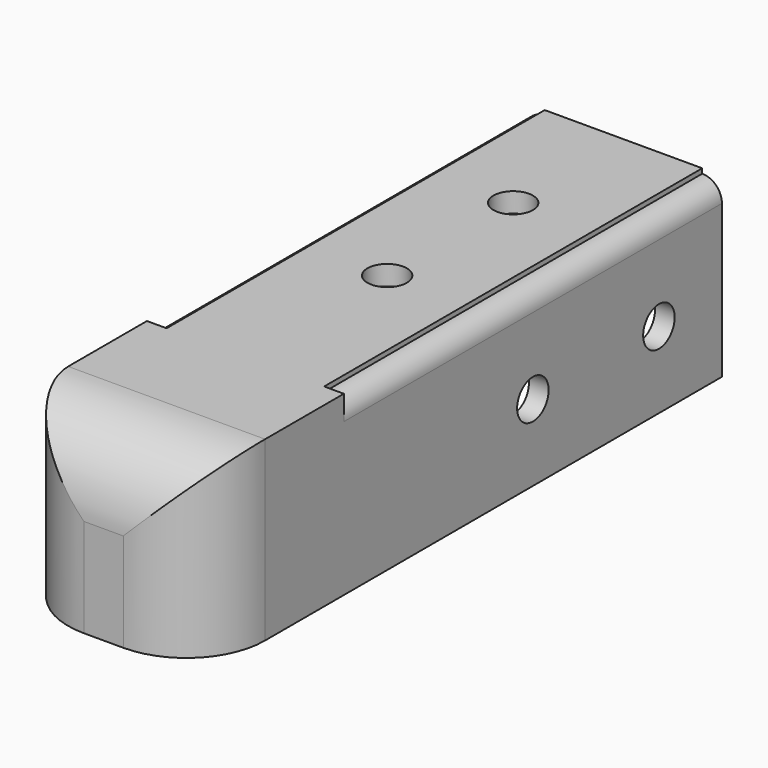
from build123d import *

# Parameters (mm, degrees)
F1_DEPTH     = 152.4
F2_W         = 50.8
F2_H         = 50.8
F3_DEPTH     = 57.15
F4_R         = 25.4
F5_T         = 5.08
F5_T3_DEPTH  = 11.7136995755
F5_T5_DEPTH  = 162.56
F5_T7_DEPTH  = 60.96
F5_T9_DEPTH  = 60.96
F5_T12_ANGLE = 90.000000001
F5_T14_ANGLE = 90.000000001
F6_R         = 6.35
F7_DEPTH     = 63.501
F8_R         = 6.35
F9_DEPTH     = 57.151


# Not quite as in the source:
# - a shell that OpenCascade refuses in one call is made with other operations: the cavity is built on its own and cut out


with BuildPart() as f1:
    # F0 (on Front) → F1 (new body)
    with BuildSketch(Plane.XZ):
        with BuildLine():
            Line((0, 49.2463004245), (0, 0))
            Line((0, 0), (6.35, 0))
            Line((6.35, 0), (6.35, 50.8))
            Line((6.35, 50.8), (57.15, 50.8))
            Line((57.15, 50.8), (57.15, 0))
            Line((57.15, 0), (63.5, 0))
            Line((63.5, 0), (63.5, 49.2463004245))
            ThreePointArc((63.5, 49.2463004245), (61.6401280605, 53.736428485), (57.15, 55.5963004245))
            Line((57.15, 55.5963004245), (57.15, 57.15))
            Line((57.15, 57.15), (6.35, 57.15))
            Line((6.35, 57.15), (6.35, 55.5963004245))
            ThreePointArc((6.35, 55.5963004245), (1.8598719395, 53.736428485), (0, 49.2463004245))
        make_face()
    extrude(amount=F1_DEPTH)

    # F2 (on face) → F3 (join)
    with BuildSketch(Plane.XZ.offset(152.4)):
        with BuildLine():
            Line((0, 49.2463004245), (0, 0))
            Line((0, 0), (6.35, 0))
            Line((6.35, 0), (6.35, 50.8))
            Line((6.35, 50.8), (57.15, 50.8))
            Line((57.15, 50.8), (57.15, 0))
            Line((57.15, 0), (63.5, 0))
            Line((63.5, 0), (63.5, 49.2463004245))
            ThreePointArc((63.5, 49.2463004245), (61.6401280605, 53.736428485), (57.15, 55.5963004245))
            Line((57.15, 55.5963004245), (57.15, 57.15))
            Line((57.15, 57.15), (6.35, 57.15))
            Line((6.35, 57.15), (6.35, 55.5963004245))
            ThreePointArc((6.35, 55.5963004245), (1.8598719395, 53.736428485), (0, 49.2463004245))
        make_face()
        with BuildLine():
            Line((0, 57.15), (0, 49.2463004245))
            ThreePointArc((0, 49.2463004245), (1.8598719395, 53.736428485), (6.35, 55.5963004245))
            Line((6.35, 55.5963004245), (6.35, 57.15))
            Line((6.35, 57.15), (0, 57.15))
        make_face()
        with BuildLine():
            ThreePointArc((57.15, 55.5963004245), (61.6401280605, 53.736428485), (63.5, 49.2463004245))
            Line((63.5, 49.2463004245), (63.5, 57.15))
            Line((63.5, 57.15), (57.15, 57.15))
            Line((57.15, 57.15), (57.15, 55.5963004245))
        make_face()
        with Locations((31.75, 25.4)):
            Rectangle(F2_W, F2_H)
    extrude(amount=F3_DEPTH)

    # F4
    f4_edges = [f1.edges().sort_by_distance(p)[0] for p in [
        (31.75, -209.55, 57.15),
        (0, -209.55, 28.575),
        (63.5, -209.55, 28.575),
    ]]
    fillet(f4_edges, radius=F4_R)

    # F5: shell of thickness 5.08, made by hand


with BuildPart() as f5_core1:
    # F5_t2: copy of F1
    add(f1.part)

    # the walls: a layer under each face that stays
    f5_faces = [f5_core1.faces().sort_by_distance(p)[0] for p in [
        (0, -92.075, 28.575),
        (31.75, -92.075, 57.15),
        (7.4394877579, -202.1105122421, 28.575),
        (1.0583333333, -152.4, 53.1981502122),
        (1.8598719395, -76.2, 53.736428485),
        (4.5357142857, 0, 4.0821428571),
        (63.5, -92.075, 28.575),
        (31.75, -202.1105122421, 49.7105122421),
        (58.2083333333, -152.4, 55.8327167374),
        (57.15, -76.2, 56.3731502122),
        (6.35, -76.2, 56.3731502122),
        (31.75, -209.55, 15.875),
        (6.35, -76.2, 25.4),
        (56.0605122421, -202.1105122421, 28.575),
        (31.75, -152.4, 25.4),
        (57.15, -76.2, 25.4),
        (31.75, -76.2, 50.8),
        (61.6401280605, -76.2, 53.736428485),
    ]]
    thicken(f5_faces, amount=-F5_T, mode=Mode.SUBTRACT)

    # F5_s4 → F5_t3 (cut)
    with BuildSketch(Plane.XY.offset(50.5163004245)):
        Polygon((6.2992, -152.3492), (6.35, -157.48), (11.43, -157.48), (11.43, -152.4), align=None)
        Polygon((57.2008, -152.3492), (57.15, -157.48), (52.07, -157.48), (52.07, -152.4), align=None)
    extrude(amount=F5_T3_DEPTH, mode=Mode.SUBTRACT)

    # F5_s6 → F5_t5 (cut)
    with BuildSketch(Plane.XZ.offset(-5.08)):
        Polygon((6.2992, 55.6471004245), (6.35, 50.5163004245), (11.43, 50.5163004245), (11.43, 55.5963004245), align=None)
        Polygon((57.2008, 55.6471004245), (52.07, 55.5963004245), (52.07, 50.5163004245), (57.15, 50.5163004245), align=None)
        Polygon((6.4008, 50.7492), (1.27, 50.8), (1.27, 55.88), (6.35, 55.88), align=None)
        Polygon((57.0992, 50.7492), (62.23, 50.8), (62.23, 55.88), (57.15, 55.88), align=None)
    extrude(amount=F5_T5_DEPTH, mode=Mode.SUBTRACT)

    # F5_s8 → F5_t7 (cut)
    with BuildSketch(Plane.XY.offset(-5.08)):
        Polygon((6.4008, -152.3492), (1.27, -152.4), (1.27, -157.48), (6.35, -157.48), align=None)
        Polygon((57.0992, -152.3492), (57.15, -157.48), (62.23, -157.48), (62.23, -152.4), align=None)
    extrude(amount=F5_T7_DEPTH, mode=Mode.SUBTRACT)

    # F5_s10 → F5_t9 (cut)
    with BuildSketch(Plane.YZ.offset(1.27)):
        Polygon((-152.3492, 50.7492), (-157.48, 50.8), (-157.48, 55.88), (-152.4, 55.88), align=None)
    extrude(amount=F5_T9_DEPTH, mode=Mode.SUBTRACT)

    # F5_s11 → F5_t12 (revolve, cut)
    with BuildSketch(Plane.YZ.offset(6.35)):
        Polygon((-152.3492, 55.6471004245), (-157.48, 55.5963004245), (-157.48, 50.5163004245), (-152.4, 50.5163004245), align=None)
    revolve(axis=Axis((6.35, -152.4, 49.2463004245), (0, -1, 0)), revolution_arc=F5_T12_ANGLE, mode=Mode.SUBTRACT)

    # F5_s13 → F5_t14 (revolve, cut)
    with BuildSketch(Plane.XY.offset(49.2463004245)):
        Polygon((63.5508, -152.3492), (63.5, -157.48), (58.42, -157.48), (58.42, -152.4), align=None)
    revolve(axis=Axis((57.15, -152.4, 49.2463004245), (0, -1, 0)), revolution_arc=F5_T14_ANGLE, mode=Mode.SUBTRACT)


with BuildPart() as f1_1:
    add(f1.part)

    # what is left inside the walls is the cavity
    f5_cavity = [f5_core1.part.solids().sort_by_distance(p)[0] for p in [
        (31.75, -157.5308, 34.713333),
    ]]
    add(f5_cavity, mode=Mode.SUBTRACT)

    # F6 (on face) → F7 (cut, through all)
    with BuildSketch(Plane(origin=(0, 0, 0), x_dir=(0, -1, 0), z_dir=(-1, 0, 0))):
        with Locations((25.4, 24.6231502122)):
            Circle(F6_R)
        with Locations((76.2, 24.6231502122)):
            Circle(F6_R)
    extrude(amount=-F7_DEPTH, mode=Mode.SUBTRACT)

    # F8 (on face) → F9 (cut, through all)
    with BuildSketch(Plane.XY.offset(57.15)):
        with Locations((31.75, -44.45)):
            Circle(F8_R)
        with Locations((31.75, -95.25)):
            Circle(F8_R)
    extrude(amount=-F9_DEPTH, mode=Mode.SUBTRACT)


solid = f1_1.part
